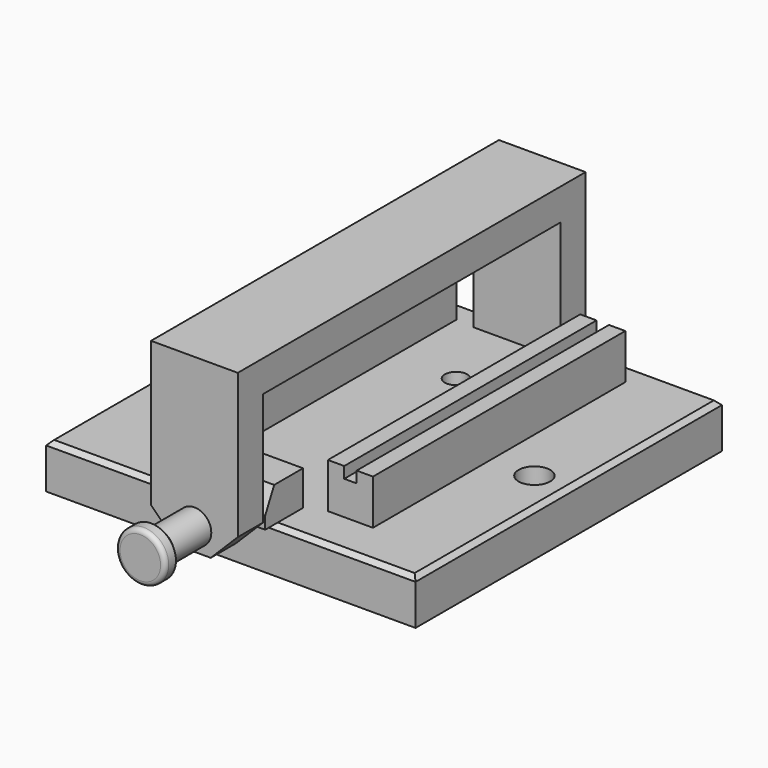
from build123d import *

# Parameters (mm, degrees)
F0_W         = 164
F0_H         = 170
F0_R         = 4.25
F0_R_2       = 5
F1_DEPTH     = 20
F3_SIZE      = 2
F4_DEPTH     = 20
F2_R         = 7
F2_R_2       = 4.25
F5_DEPTH     = 9
F6_W         = 20
F6_H         = 140
F7_DEPTH     = 20
F8_W         = 5.5
F8_H         = 140
F9_DEPTH     = 5
F10_W        = 38.5
F10_H        = 2.8
F10_H_2      = 11.2
F11_DEPTH    = 67.5
F12_W        = 38.5
F12_H        = 14
F13_DEPTH    = 179
F14_W        = 38.5
F14_H        = 14
F15_DEPTH    = 62.2
F16_SIZE     = 12
F17_R        = 4.5
F18_DEPTH    = 14
F19_R        = 7.5
F19_R_2      = 4.5
F20_DEPTH    = 19
F21_R        = 11
F21_R_2      = 7.5
F22_DEPTH    = 11
F23_S5_R     = 7.5
F23_T6_DEPTH = 17
F24_R        = 2
F25_W        = 38.5
F25_H        = 16
F25_H_2      = 5
F26_DEPTH    = 15.5
F27_SIZE2    = 5
F27_SIZE     = 10


# Not quite as in the source:
# - a fillet or chamfer that OpenCascade refuses, or shapes differently, is made with other operations: its cross-section is extruded or revolved along the edge and cut away or added


with BuildPart() as f1:
    # F0 (on Top) → F1 (new body)
    with BuildSketch(Plane.XY):
        Rectangle(F0_W, F0_H)
        with Locations((-66.75, 0)):
            Circle(F0_R, mode=Mode.SUBTRACT)
        with Locations((0, 40)):
            Circle(F0_R_2, mode=Mode.SUBTRACT)
        with Locations((66.75, 0)):
            Circle(F0_R, mode=Mode.SUBTRACT)
    extrude(amount=F1_DEPTH)

    # F3
    f3_edges = [f1.edges().sort_by_distance(p)[0] for p in [
        (82, 0, 20),
        (0, -85, 20),
        (0, 85, 20),
        (-82, 0, 20),
    ]]
    chamfer(f3_edges, length=F3_SIZE)

    # F0 (on Top) → F4 (cut)
    with BuildSketch(Plane.XY):
        with Locations((0, 40)):
            Circle(F0_R_2)
    extrude(amount=F4_DEPTH, mode=Mode.SUBTRACT)

    # F2 (on face) → F5 (cut)
    with BuildSketch(Plane.XY.offset(20)):
        with Locations((-66.75, 0)):
            Circle(F2_R)
        with Locations((-66.75, 0)):
            Circle(F2_R_2, mode=Mode.SUBTRACT)
        with Locations((66.75, 0)):
            Circle(F2_R)
        with Locations((66.75, 0)):
            Circle(F2_R_2, mode=Mode.SUBTRACT)
    extrude(amount=-F5_DEPTH, mode=Mode.SUBTRACT)

    # F6 (on face) → F7 (join)
    with BuildSketch(Plane.XY.offset(20)):
        with Locations((-37.5, 4.5)):
            Rectangle(F6_W, F6_H)
        with Locations((37.5, 4.5)):
            Rectangle(F6_W, F6_H)
    extrude(amount=F7_DEPTH)

    # F8 (on face) → F9 (cut)
    with BuildSketch(Plane.XY.offset(40)):
        with Locations((-37.5, 4.5)):
            Rectangle(F8_W, F8_H)
        with Locations((37.5, 4.5)):
            Rectangle(F8_W, F8_H)
    extrude(amount=-F9_DEPTH, mode=Mode.SUBTRACT)

    # F10 (on face) → F11 (join)
    with BuildSketch(Plane.XY.offset(20)):
        with Locations((0, 86.4)):
            Rectangle(F10_W, F10_H)
        with Locations((0, 79.4)):
            Rectangle(F10_W, F10_H_2)
    extrude(amount=F11_DEPTH)

    # F12 (on face) → F13 (join)
    with BuildSketch(Plane.XZ.offset(-73.8)):
        with Locations((0, 80.5)):
            Rectangle(F12_W, F12_H)
    extrude(amount=F13_DEPTH)

    # F14 (on face) → F15 (join)
    with BuildSketch(Plane(origin=(0, 0, 73.5), x_dir=(1, 0, 0), z_dir=(0, 0, -1))):
        with Locations((0, 98.2)):
            Rectangle(F14_W, F14_H)
    extrude(amount=F15_DEPTH)

    # F16
    f16_edges = [f1.edges().sort_by_distance(p)[0] for p in [
        (-19.25, -98.2, 11.3),
        (19.25, -98.2, 11.3),
    ]]
    chamfer(f16_edges, length=F16_SIZE)

    # F17 (on face) → F18 (cut)
    with BuildSketch(Plane.XZ.offset(105.2)):
        with Locations((0, 21.2)):
            Circle(F17_R)
    extrude(amount=-F18_DEPTH, mode=Mode.SUBTRACT)

    # F19 (on face) → F20 (join)
    with BuildSketch(Plane.XZ.offset(105.2)):
        with Locations((0, 21.2)):
            Circle(F19_R)
        with Locations((0, 21.2)):
            Circle(F19_R_2, mode=Mode.SUBTRACT)
        with Locations((0, 21.2)):
            Circle(F19_R_2)
    extrude(amount=F20_DEPTH)

    # F21 (on face) → F22 (join)
    with BuildSketch(Plane.XZ.offset(124.2)):
        with Locations((0, 21.2)):
            Circle(F21_R)
        with Locations((0, 21.2)):
            Circle(F21_R_2, mode=Mode.SUBTRACT)
        with Locations((0, 21.2)):
            Circle(F21_R_2)
    extrude(amount=F22_DEPTH)

    # F23: chamfer of 5 on 1 edges, made by hand


with BuildPart() as f23_tool2:
    # F23_s3 → F23_t4 (revolve)
    with BuildSketch(Plane.XY.offset(21.2)):
        Polygon((11, -129.2), (6, -124.2), (11, -124.2), align=None)
    revolve(axis=Axis((0, -124.2, 21.2), (0, -1, 0)))

    # F23_s5 → F23_t6 (cut, symmetric)
    with BuildSketch(Plane.XZ.offset(126.7)):
        with Locations((0, 21.2)):
            Circle(F23_S5_R)
    extrude(amount=F23_T6_DEPTH, both=True, mode=Mode.SUBTRACT)


with BuildPart() as f1_1:
    add(f1.part)

    # F23_t1: cut F23_tool2
    add(f23_tool2.part, mode=Mode.SUBTRACT)

    # F24
    f24_edges = [f1_1.edges().sort_by_distance(p)[0] for p in [
        (-11, -135.2, 21.2),
    ]]
    fillet(f24_edges, radius=F24_R)

    # F25 (on face) → F26 (join)
    with BuildSketch(Plane.XY.offset(20)):
        with Locations((0, -77)):
            Rectangle(F25_W, F25_H)
        with Locations((0, -87.5)):
            Rectangle(F25_W, F25_H_2)
    extrude(amount=F26_DEPTH)

    # F27
    f27_edges = [f1_1.edges().sort_by_distance(p)[0] for p in [
        (0, -90, 35.5),
    ]]
    f27_side = f1_1.faces().sort_by_distance((0, -90, 27.75))[0]
    chamfer(f27_edges, length=F27_SIZE, length2=F27_SIZE2, reference=f27_side)


solid = f1_1.part
